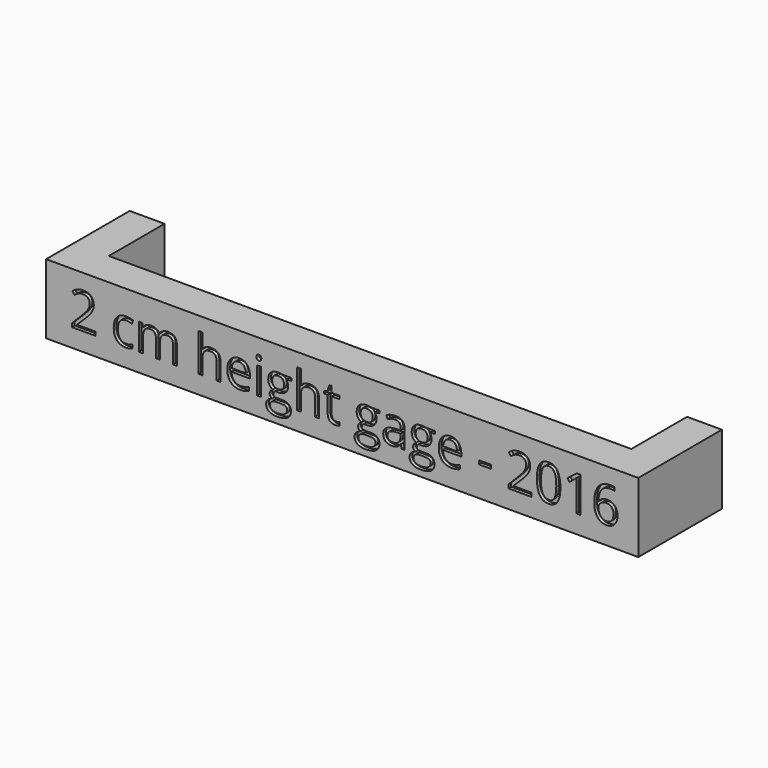
from build123d import *

# Parameters (mm, degrees)
F1_DEPTH     = 20
F2_TEXT_SIZE = 14.3102952279
F3_DEPTH     = 1


# Not quite as in the source:
# - Text() gives the source's letters only with a copy of the font that has no kerning and outlines rounded to 1/6400 em; it was checked with that copy


with BuildPart() as f1:
    # F0 (on Top) → F1 (new body)
    with BuildSketch(Plane.XY):
        Polygon((10, 30), (0, 30), (0, 0), (170, 0), (170, 30), (160, 30), (160, 10), (10, 10), align=None)
    extrude(amount=F1_DEPTH)

    # F2 (on face) → F3 (cut)
    with BuildSketch(Plane.XZ):
        with Locations((6.7154197022, 5.2319206297)):
            Text('2 cm height gage - 2016', F2_TEXT_SIZE, font='Open Sans', text_align=(TextAlign.LEFT, TextAlign.BOTTOM))
    extrude(amount=-F3_DEPTH, mode=Mode.SUBTRACT)


solid = f1.part
